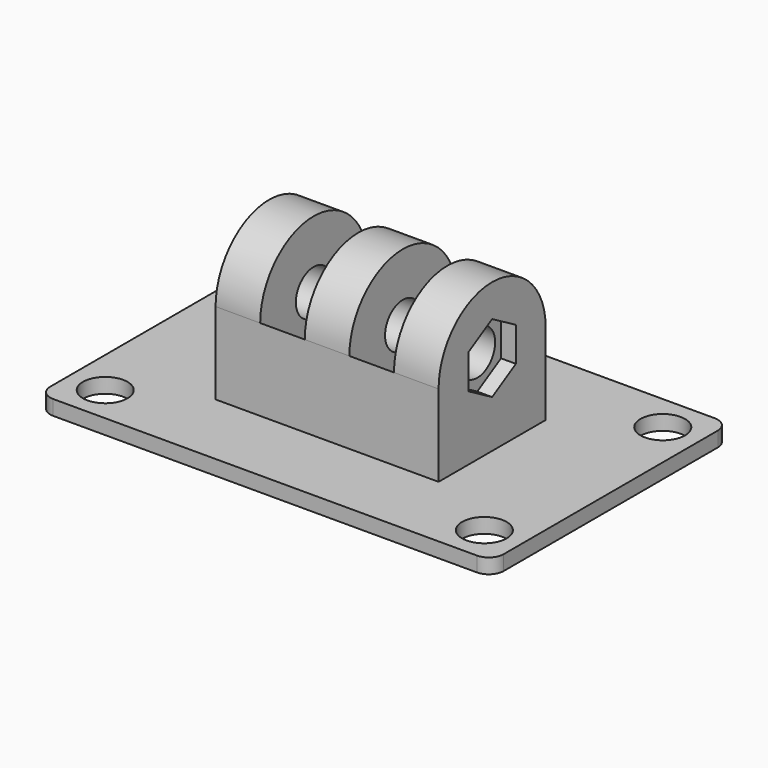
from build123d import *

# Parameters (mm, degrees)
F0_R      = 3
F1_DEPTH  = 2
F2_W      = 30
F2_H      = 18
F3_DEPTH  = 20
F6_DEPTH  = 30
F7_R      = 9
F8_DEPTH  = 30
F10_R     = 9
F11_DEPTH = 6
F13_START = 6
F12_R     = 9
F13_DEPTH = 12
F14_DEPTH = 6
F15_DEPTH = 6
F16_R     = 3
F17_DEPTH = 30
F18_R     = 3
F19_DEPTH = 2


# Not quite as in the source:
# - a feature names something its author has since deleted; it is built from what else it names


with BuildPart() as f1:
    # F0 (on Top) → F1 (new body)
    with BuildSketch(Plane.XY):
        with BuildLine():
            Line((28.6193578921, 20.4223022205), (-28.3806421079, 20.4223022205))
            ThreePointArc((-28.3806421079, 20.4223022205), (-29.7948556703, 19.8365157828), (-30.3806421079, 18.4223022205))
            Line((-30.3806421079, 18.4223022205), (-30.3806421079, -17.5776977795))
            ThreePointArc((-30.3806421079, -17.5776977795), (-29.7948556703, -18.9919113419), (-28.3806421079, -19.5776977795))
            Line((-28.3806421079, -19.5776977795), (28.6193578921, -19.5776977795))
            ThreePointArc((28.6193578921, -19.5776977795), (30.0335714544, -18.9919113419), (30.6193578921, -17.5776977795))
            Line((30.6193578921, -17.5776977795), (30.6193578921, 18.4223022205))
            ThreePointArc((30.6193578921, 18.4223022205), (30.0335714544, 19.8365157828), (28.6193578921, 20.4223022205))
        make_face()
        with Locations((-25.3806421079, -14.5776977795)):
            Circle(F0_R, mode=Mode.SUBTRACT)
        with Locations((25.6193578921, -14.5776977795)):
            Circle(F0_R, mode=Mode.SUBTRACT)
        with Locations((-25.3806421079, 15.4223022205)):
            Circle(F0_R, mode=Mode.SUBTRACT)
        with Locations((25.6193578921, 15.4223022205)):
            Circle(F0_R, mode=Mode.SUBTRACT)
    extrude(amount=F1_DEPTH)

    # F2 (on face) → F3 (join)
    with BuildSketch(Plane.XY.offset(2)):
        Rectangle(F2_W, F2_H)
    extrude(amount=F3_DEPTH)

    # F5 (on face) + F4 (on face) → F6 (cut)
    with BuildSketch(Plane(origin=(-15, 0, 0), x_dir=(0, -1, 0), z_dir=(-1, 0, 0))):
        with BuildLine():
            Line((9, 22), (0, 22))
            ThreePointArc((0, 22), (6.3639610307, 19.3639610307), (9, 13))
            Line((9, 13), (9, 22))
        make_face()
    with BuildSketch(Plane(origin=(-15, 0, 0), x_dir=(0, -1, 0), z_dir=(-1, 0, 0))):
        with BuildLine():
            ThreePointArc((-9, 13), (-6.3639610307, 19.3639610307), (0, 22))
            Line((0, 22), (-9, 22))
            Line((-9, 22), (-9, 13))
        make_face()
    extrude(amount=-F6_DEPTH, mode=Mode.SUBTRACT)

    # F7 (on face) → F8 (cut)
    with BuildSketch(Plane(origin=(-15, 0, 0), x_dir=(0, -1, 0), z_dir=(-1, 0, 0))):
        with Locations((0, 13)):
            Circle(F7_R)
    extrude(amount=-F8_DEPTH, mode=Mode.SUBTRACT)

    # F10 (on face) → F11 (join)
    with BuildSketch(Plane.YZ.offset(15)):
        with Locations((0, 13)):
            Circle(F10_R)
    extrude(amount=-F11_DEPTH)

    # F12 (on face) → F13 (join)
    with BuildSketch(Plane(origin=(9, 0, 0), x_dir=(0, -1, 0), z_dir=(-1, 0, 0)).offset(F13_START)):
        with Locations((0, 13)):
            Circle(F12_R)
    extrude(amount=F13_DEPTH)

    # F14 (cut): a face of the model
    f14_faces = [f1.faces().sort_by_distance(p)[0] for p in [
        (-9, 0, 13),
    ]]
    extrude(f14_faces, amount=-F14_DEPTH, mode=Mode.SUBTRACT)


with BuildPart() as f15:
    # F9 (on face) → F15 (new body)
    with BuildSketch(Plane(origin=(-15, 0, 0), x_dir=(0, -1, 0), z_dir=(-1, 0, 0))):
        with BuildLine():
            ThreePointArc((-9, 13), (0, 4), (9, 13))
            ThreePointArc((9, 13), (0, 22), (-9, 13))
        make_face()
    extrude(amount=-F15_DEPTH)


with BuildPart() as f17_tool:
    # F16 (on face) → F17 (new body)
    with BuildSketch(Plane(origin=(-15, 0, 0), x_dir=(0, -1, 0), z_dir=(-1, 0, 0))):
        with Locations((0, 13)):
            Circle(F16_R)
    extrude(amount=-F17_DEPTH)


with BuildPart() as f1_1:
    add(f1.part)

    # F17: cut by f17_tool
    add(f17_tool.part, mode=Mode.SUBTRACT)

    # F18 (on face) → F19 (cut)
    with BuildSketch(Plane.YZ.offset(15)):
        Polygon((4, 10.6905989232), (4, 15.3094010768), (0, 17.6188021535), (-4, 15.3094010768), (-4, 10.6905989232), (0, 8.3811978465), align=None)
        with Locations((0, 13)):
            Circle(F18_R, mode=Mode.SUBTRACT)
    extrude(amount=-F19_DEPTH, mode=Mode.SUBTRACT)


with BuildPart() as f15_1:
    add(f15.part)

    # F17: cut by f17_tool
    add(f17_tool.part, mode=Mode.SUBTRACT)


solid = Compound([f1_1.part, f15_1.part])
